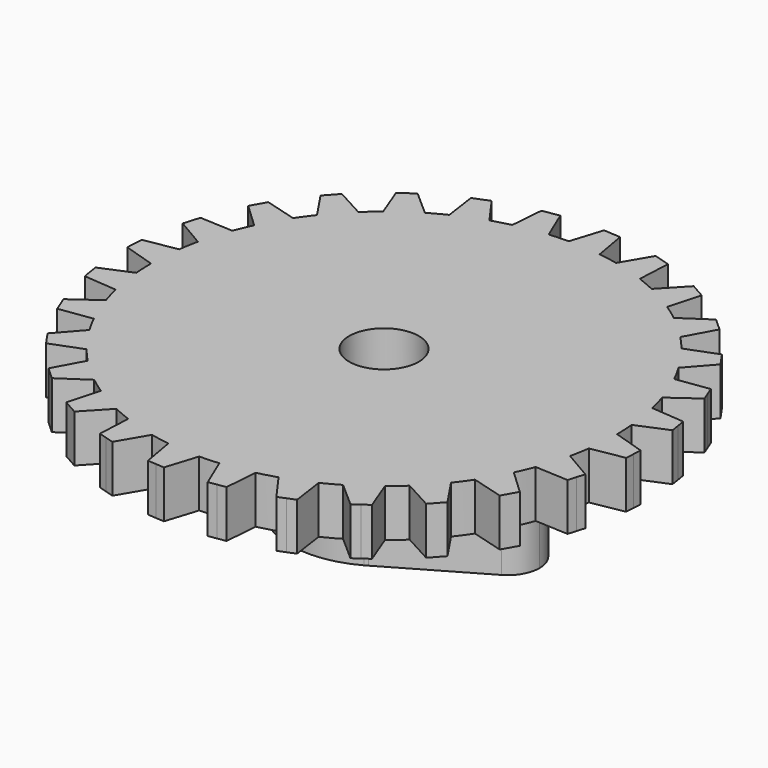
from build123d import *

# Parameters (mm, degrees)
F0_R     = 3.3
F1_DEPTH = 4.5
F2_DEPTH = 9
F4_COUNT = 28
F5_DEPTH = 9


# Not quite as in the source:
# - a feature names something its author has since deleted; it is built from what else it names


with BuildPart() as f1:
    # F0 (on Top) → F1 (new body)
    with BuildSketch(Plane.XY):
        with BuildLine():
            ThreePointArc((21.7954284513, -2.9932087503), (21.9487975289, -1.5000956754), (22, 0))
            ThreePointArc((22, 0), (21.9999455382, 0.0489521697), (21.9997821532, 0.097904097))
            ThreePointArc((21.9997821532, 0.097904097), (21.9765398394, 1.0157247108), (21.9150231618, 1.9317763373))
            ThreePointArc((21.9150231618, 1.9317763373), (21.7246308845, 3.4699298167), (21.426415972, 4.9908615085))
            ThreePointArc((21.426415972, 4.9908615085), (21.1995220913, 5.8804985418), (20.9357071018, 6.759894093))
            ThreePointArc((20.9357071018, 6.759894093), (20.4078170076, 8.2171165859), (19.778639825, 9.6335562839))
            ThreePointArc((19.778639825, 9.6335562839), (19.3594717841, 10.4503996211), (18.9065872678, 11.249042532))
            ThreePointArc((18.9065872678, 11.249042532), (18.0676699703, 12.5522628177), (17.1390800887, 13.793184321))
            ThreePointArc((17.1390800887, 13.793184321), (16.5486567235, 14.4962740264), (15.9294122011, 15.1741170065))
            ThreePointArc((15.9294122011, 15.1741170065), (14.8215345166, 16.2579861782), (13.6400953103, 17.2611645009))
            ThreePointArc((13.6400953103, 17.2611645009), (12.9080229136, 17.8152447208), (12.1534698913, 18.3382978927))
            ThreePointArc((12.1534698913, 18.3382978927), (10.832185433, 19.1484662243), (9.4571391969, 19.8635978164))
            ThreePointArc((9.4571391969, 19.8635978164), (8.6201269356, 20.2408846549), (7.7681018526, 20.5829199485))
            ThreePointArc((7.7681018526, 20.5829199485), (6.2996653405, 21.0787622169), (4.7999626346, 21.4699873942))
            ThreePointArc((4.7999626346, 21.4699873942), (3.8999817986, 21.6515621139), (2.9932087503, 21.7954284513))
            ThreePointArc((2.9932087503, 21.7954284513), (1.4512537227, 21.9520810547), (-0.097904097, 21.9997821532))
            ThreePointArc((-0.097904097, 21.9997821532), (-1.0157247108, 21.9765398394), (-1.9317763373, 21.9150231618))
            ThreePointArc((-1.9317763373, 21.9150231618), (-3.4699298167, 21.7246308845), (-4.9908615085, 21.426415972))
            ThreePointArc((-4.9908615085, 21.426415972), (-5.8804985418, 21.1995220913), (-6.759894093, 20.9357071018))
            ThreePointArc((-6.759894093, 20.9357071018), (-8.2171165859, 20.4078170076), (-9.6335562839, 19.778639825))
            ThreePointArc((-9.6335562839, 19.778639825), (-10.4503996211, 19.3594717841), (-11.249042532, 18.9065872678))
            ThreePointArc((-11.249042532, 18.9065872678), (-12.5522628177, 18.0676699703), (-13.793184321, 17.1390800887))
            ThreePointArc((-13.793184321, 17.1390800887), (-14.4962740264, 16.5486567235), (-15.1741170065, 15.9294122011))
            ThreePointArc((-15.1741170065, 15.9294122011), (-16.2579861782, 14.8215345166), (-17.2611645009, 13.6400953103))
            ThreePointArc((-17.2611645009, 13.6400953103), (-17.8152447208, 12.9080229136), (-18.3382978927, 12.1534698913))
            ThreePointArc((-18.3382978927, 12.1534698913), (-19.1484662243, 10.832185433), (-19.8635978164, 9.4571391969))
            ThreePointArc((-19.8635978164, 9.4571391969), (-20.2408846549, 8.6201269356), (-20.5829199485, 7.7681018526))
            ThreePointArc((-20.5829199485, 7.7681018526), (-21.0787622169, 6.2996653405), (-21.4699873942, 4.7999626346))
            ThreePointArc((-21.4699873942, 4.7999626346), (-21.6515621139, 3.8999817986), (-21.7954284513, 2.9932087503))
            ThreePointArc((-21.7954284513, 2.9932087503), (-21.9520810547, 1.4512537227), (-21.9997821532, -0.097904097))
            ThreePointArc((-21.9997821532, -0.097904097), (-21.9765398394, -1.0157247108), (-21.9150231618, -1.9317763373))
            ThreePointArc((-21.9150231618, -1.9317763373), (-21.7246308845, -3.4699298167), (-21.426415972, -4.9908615085))
            ThreePointArc((-21.426415972, -4.9908615085), (-21.1995220913, -5.8804985418), (-20.9357071018, -6.759894093))
            ThreePointArc((-20.9357071018, -6.759894093), (-20.4078170076, -8.2171165859), (-19.778639825, -9.6335562839))
            ThreePointArc((-19.778639825, -9.6335562839), (-19.3594717841, -10.4503996211), (-18.9065872678, -11.249042532))
            ThreePointArc((-18.9065872678, -11.249042532), (-18.0676699703, -12.5522628177), (-17.1390800887, -13.793184321))
            ThreePointArc((-17.1390800887, -13.793184321), (-16.5486567235, -14.4962740264), (-15.9294122011, -15.1741170065))
            ThreePointArc((-15.9294122011, -15.1741170065), (-14.8215345166, -16.2579861782), (-13.6400953103, -17.2611645009))
            ThreePointArc((-13.6400953103, -17.2611645009), (-12.9080229136, -17.8152447208), (-12.1534698913, -18.3382978927))
            ThreePointArc((-12.1534698913, -18.3382978927), (-10.832185433, -19.1484662243), (-9.4571391969, -19.8635978164))
            ThreePointArc((-9.4571391969, -19.8635978164), (-8.6201269356, -20.2408846549), (-7.7681018526, -20.5829199485))
            ThreePointArc((-7.7681018526, -20.5829199485), (-6.2996653405, -21.0787622169), (-4.7999626346, -21.4699873942))
            ThreePointArc((-4.7999626346, -21.4699873942), (-3.8999817986, -21.6515621139), (-2.9932087503, -21.7954284513))
            ThreePointArc((-2.9932087503, -21.7954284513), (-1.4512537227, -21.9520810547), (0.097904097, -21.9997821532))
            ThreePointArc((0.097904097, -21.9997821532), (1.0157247108, -21.9765398394), (1.9317763373, -21.9150231618))
            ThreePointArc((1.9317763373, -21.9150231618), (3.4699298167, -21.7246308845), (4.9908615085, -21.426415972))
            ThreePointArc((4.9908615085, -21.426415972), (5.8804985418, -21.1995220913), (6.759894093, -20.9357071018))
            ThreePointArc((6.759894093, -20.9357071018), (8.2171165859, -20.4078170076), (9.6335562839, -19.778639825))
            ThreePointArc((9.6335562839, -19.778639825), (10.4503996211, -19.3594717841), (11.249042532, -18.9065872678))
            ThreePointArc((11.249042532, -18.9065872678), (12.5522628177, -18.0676699703), (13.793184321, -17.1390800887))
            ThreePointArc((13.793184321, -17.1390800887), (14.4962740264, -16.5486567235), (15.1741170065, -15.9294122011))
            ThreePointArc((15.1741170065, -15.9294122011), (16.2579861782, -14.8215345166), (17.2611645009, -13.6400953103))
            ThreePointArc((17.2611645009, -13.6400953103), (17.8152447208, -12.9080229136), (18.3382978927, -12.1534698913))
            ThreePointArc((18.3382978927, -12.1534698913), (19.1484662243, -10.832185433), (19.8635978164, -9.4571391969))
            ThreePointArc((19.8635978164, -9.4571391969), (20.2408846549, -8.6201269356), (20.5829199485, -7.7681018526))
            ThreePointArc((20.5829199485, -7.7681018526), (21.0787622169, -6.2996653405), (21.4699873942, -4.7999626346))
            ThreePointArc((21.4699873942, -4.7999626346), (21.6515621139, -3.8999817986), (21.7954284513, -2.9932087503))
        make_face()
        with BuildLine():
            ThreePointArc((4.2957761194, -7.7649288031), (-8.8739963819, 0), (4.2957761194, 7.7649288031))
            ThreePointArc((4.2957761194, 7.7649288031), (4.4440805495, 7.6810129446), (4.5907463478, 7.5942649253))
            Line((4.5907463478, 7.5942649253), (13.2283979256, 2.5966923855))
            ThreePointArc((13.2283979256, 2.5966923855), (14.3247709146, 1.4988023682), (14.7260036181, 0))
            ThreePointArc((14.7260036181, 0), (14.3247709146, -1.4988023682), (13.2283979256, -2.5966923855))
            Line((13.2283979256, -2.5966923855), (4.5907463478, -7.5942649253))
            ThreePointArc((4.5907463478, -7.5942649253), (4.4440805495, -7.6810129446), (4.2957761194, -7.7649288031))
        make_face(mode=Mode.SUBTRACT)
        with BuildLine():
            Line((4.5907463478, 7.5942649253), (4.2957761194, 7.7649288031))
            ThreePointArc((4.2957761194, 7.7649288031), (-8.8739963819, 0), (4.2957761194, -7.7649288031))
            Line((4.2957761194, -7.7649288031), (4.5907463478, -7.5942649253))
            ThreePointArc((4.5907463478, -7.5942649253), (7.5224602815, -4.7074837333), (8.8370675717, -0.8087326625))
            ThreePointArc((8.8370675717, -0.8087326625), (8.7260036181, 0), (8.8370675717, 0.8087326625))
            ThreePointArc((8.8370675717, 0.8087326625), (7.5224602815, 4.7074837333), (4.5907463478, 7.5942649253))
        make_face()
        Circle(F0_R, mode=Mode.SUBTRACT)
        with BuildLine():
            Line((13.2283979256, 2.5966923855), (4.5907463478, 7.5942649253))
            ThreePointArc((4.5907463478, 7.5942649253), (7.5224602815, 4.7074837333), (8.8370675717, 0.8087326625))
            ThreePointArc((8.8370675717, 0.8087326625), (10.5947103355, 2.7785203812), (13.2283979256, 2.5966923855))
        make_face()
        with BuildLine():
            ThreePointArc((8.8370675717, -0.8087326625), (7.5224602815, -4.7074837333), (4.5907463478, -7.5942649253))
            Line((4.5907463478, -7.5942649253), (13.2283979256, -2.5966923855))
            ThreePointArc((13.2283979256, -2.5966923855), (10.5947103355, -2.7785203812), (8.8370675717, -0.8087326625))
        make_face()
        with BuildLine():
            ThreePointArc((-9.6335562839, 19.778639825), (-8.2171165859, 20.4078170076), (-6.759894093, 20.9357071018))
            Line((-6.759894093, 20.9357071018), (-8.5955300473, 23.4895053845))
            Line((-8.5955300473, 23.4895053845), (-9.3376324839, 23.190701145))
            Line((-9.3376324839, 23.190701145), (-10.0797349206, 22.8918969055))
            Line((-10.0797349206, 22.8918969055), (-9.6335562839, 19.778639825))
        make_face()
        with BuildLine():
            ThreePointArc((-17.2611645009, 13.6400953103), (-16.2579861782, 14.8215345166), (-15.1741170065, 15.9294122011))
            Line((-15.1741170065, 15.9294122011), (-17.936019402, 17.4338523572))
            Line((-17.936019402, 17.4338523572), (-18.4749842935, 16.8426528598))
            Line((-18.4749842935, 16.8426528598), (-19.013949185, 16.2514533624))
            Line((-19.013949185, 16.2514533624), (-17.2611645009, 13.6400953103))
        make_face()
        with BuildLine():
            ThreePointArc((17.1390800887, 13.793184321), (18.0676699703, 12.5522628177), (18.9065872678, 11.249042532))
            Line((18.9065872678, 11.249042532), (20.9878890687, 13.6069288394))
            Line((20.9878890687, 13.6069288394), (20.531443148, 14.2639350202))
            Line((20.531443148, 14.2639350202), (20.0749972274, 14.9209412009))
            Line((20.0749972274, 14.9209412009), (17.1390800887, 13.793184321))
        make_face()
        with BuildLine():
            ThreePointArc((-21.4699873942, 4.7999626346), (-21.0787622169, 6.2996653405), (-20.5829199485, 7.7681018526))
            Line((-20.5829199485, 7.7681018526), (-23.7240601432, 7.9252110584))
            Line((-23.7240601432, 7.9252110584), (-23.9531388829, 7.1587106142))
            Line((-23.9531388829, 7.1587106142), (-24.1822176225, 6.3922101699))
            Line((-24.1822176225, 6.3922101699), (-21.4699873942, 4.7999626346))
        make_face()
        with BuildLine():
            ThreePointArc((19.778639825, 9.6335562839), (20.4078170076, 8.2171165859), (20.9357071018, 6.759894093))
            Line((20.9357071018, 6.759894093), (23.4895053845, 8.5955300473))
            Line((23.4895053845, 8.5955300473), (23.190701145, 9.3376324839))
            Line((23.190701145, 9.3376324839), (22.8918969055, 10.0797349206))
            Line((22.8918969055, 10.0797349206), (19.778639825, 9.6335562839))
        make_face()
        with BuildLine():
            Line((-0.8508944647, -24.9983195157), (0.097904097, -21.9997821532))
            ThreePointArc((0.097904097, -21.9997821532), (-1.4512537227, -21.9520810547), (-2.9932087503, -21.7954284513))
            Line((-2.9932087503, -21.7954284513), (-2.4474094505, -24.8927737904))
            Line((-2.4474094505, -24.8927737904), (-1.6491519576, -24.9455466531))
            Line((-1.6491519576, -24.9455466531), (-0.8508944647, -24.9983195157))
        make_face()
        with BuildLine():
            ThreePointArc((21.426415972, 4.9908615085), (21.7246308845, 3.4699298167), (21.9150231618, 1.9317763373))
            Line((21.9150231618, 1.9317763373), (24.8132598166, 3.1531154868))
            Line((24.8132598166, 3.1531154868), (24.6870805506, 3.9431020644))
            Line((24.6870805506, 3.9431020644), (24.5609012845, 4.733088642))
            Line((24.5609012845, 4.733088642), (21.426415972, 4.9908615085))
        make_face()
        with BuildLine():
            Line((19.013949185, -16.2514533624), (17.2611645009, -13.6400953103))
            ThreePointArc((17.2611645009, -13.6400953103), (16.2579861782, -14.8215345166), (15.1741170065, -15.9294122011))
            Line((15.1741170065, -15.9294122011), (17.936019402, -17.4338523572))
            Line((17.936019402, -17.4338523572), (18.4749842935, -16.8426528598))
            Line((18.4749842935, -16.8426528598), (19.013949185, -16.2514533624))
        make_face()
        with BuildLine():
            Line((-20.0749972274, -14.9209412009), (-17.1390800887, -13.793184321))
            ThreePointArc((-17.1390800887, -13.793184321), (-18.0676699703, -12.5522628177), (-18.9065872678, -11.249042532))
            Line((-18.9065872678, -11.249042532), (-20.9878890687, -13.6069288394))
            Line((-20.9878890687, -13.6069288394), (-20.531443148, -14.2639350202))
            Line((-20.531443148, -14.2639350202), (-20.0749972274, -14.9209412009))
        make_face()
        with BuildLine():
            Line((-22.8918969055, -10.0797349206), (-19.778639825, -9.6335562839))
            ThreePointArc((-19.778639825, -9.6335562839), (-20.4078170076, -8.2171165859), (-20.9357071018, -6.759894093))
            Line((-20.9357071018, -6.759894093), (-23.4895053845, -8.5955300473))
            Line((-23.4895053845, -8.5955300473), (-23.190701145, -9.3376324839))
            Line((-23.190701145, -9.3376324839), (-22.8918969055, -10.0797349206))
        make_face()
        with BuildLine():
            Line((-24.5609012845, -4.733088642), (-21.426415972, -4.9908615085))
            ThreePointArc((-21.426415972, -4.9908615085), (-21.7246308845, -3.4699298167), (-21.9150231618, -1.9317763373))
            Line((-21.9150231618, -1.9317763373), (-24.8132598166, -3.1531154868))
            Line((-24.8132598166, -3.1531154868), (-24.6870805506, -3.9431020644))
            Line((-24.6870805506, -3.9431020644), (-24.5609012845, -4.733088642))
        make_face()
        with BuildLine():
            Line((-16.2514533624, -19.013949185), (-13.6400953103, -17.2611645009))
            ThreePointArc((-13.6400953103, -17.2611645009), (-14.8215345166, -16.2579861782), (-15.9294122011, -15.1741170065))
            Line((-15.9294122011, -15.1741170065), (-17.4338523572, -17.936019402))
            Line((-17.4338523572, -17.936019402), (-16.8426528598, -18.4749842935))
            Line((-16.8426528598, -18.4749842935), (-16.2514533624, -19.013949185))
        make_face()
        with BuildLine():
            ThreePointArc((-13.793184321, 17.1390800887), (-12.5522628177, 18.0676699703), (-11.249042532, 18.9065872678))
            Line((-11.249042532, 18.9065872678), (-13.6069288394, 20.9878890687))
            Line((-13.6069288394, 20.9878890687), (-14.2639350202, 20.531443148))
            Line((-14.2639350202, 20.531443148), (-14.9209412009, 20.0749972274))
            Line((-14.9209412009, 20.0749972274), (-13.793184321, 17.1390800887))
        make_face()
        with BuildLine():
            Line((-11.6129937657, -22.1535183616), (-9.4571391969, -19.8635978164))
            ThreePointArc((-9.4571391969, -19.8635978164), (-10.832185433, -19.1484662243), (-12.1534698913, -18.3382978927))
            Line((-12.1534698913, -18.3382978927), (-13.0056094911, -21.3657230574))
            Line((-13.0056094911, -21.3657230574), (-12.3093016284, -21.7596207095))
            Line((-12.3093016284, -21.7596207095), (-11.6129937657, -22.1535183616))
        make_face()
        with BuildLine():
            Line((14.9209412009, -20.0749972274), (13.793184321, -17.1390800887))
            ThreePointArc((13.793184321, -17.1390800887), (12.5522628177, -18.0676699703), (11.249042532, -18.9065872678))
            Line((11.249042532, -18.9065872678), (13.6069288394, -20.9878890687))
            Line((13.6069288394, -20.9878890687), (14.2639350202, -20.531443148))
            Line((14.2639350202, -20.531443148), (14.9209412009, -20.0749972274))
        make_face()
        with BuildLine():
            ThreePointArc((-21.9997821532, -0.097904097), (-21.9520810547, 1.4512537227), (-21.7954284513, 2.9932087503))
            Line((-21.7954284513, 2.9932087503), (-24.8927737904, 2.4474094505))
            Line((-24.8927737904, 2.4474094505), (-24.9455466531, 1.6491519576))
            Line((-24.9455466531, 1.6491519576), (-24.9983195157, 0.8508944647))
            Line((-24.9983195157, 0.8508944647), (-21.9997821532, -0.097904097))
        make_face()
        with BuildLine():
            ThreePointArc((13.6400953103, 17.2611645009), (14.8215345166, 16.2579861782), (15.9294122011, 15.1741170065))
            Line((15.9294122011, 15.1741170065), (17.4338523572, 17.936019402))
            Line((17.4338523572, 17.936019402), (16.8426528598, 18.4749842935))
            Line((16.8426528598, 18.4749842935), (16.2514533624, 19.013949185))
            Line((16.2514533624, 19.013949185), (13.6400953103, 17.2611645009))
        make_face()
        with BuildLine():
            Line((22.1535183616, -11.6129937657), (19.8635978164, -9.4571391969))
            ThreePointArc((19.8635978164, -9.4571391969), (19.1484662243, -10.832185433), (18.3382978927, -12.1534698913))
            Line((18.3382978927, -12.1534698913), (21.3657230574, -13.0056094911))
            Line((21.3657230574, -13.0056094911), (21.7596207095, -12.3093016284))
            Line((21.7596207095, -12.3093016284), (22.1535183616, -11.6129937657))
        make_face()
        with BuildLine():
            Line((4.733088642, -24.5609012845), (4.9908615085, -21.426415972))
            ThreePointArc((4.9908615085, -21.426415972), (3.4699298167, -21.7246308845), (1.9317763373, -21.9150231618))
            Line((1.9317763373, -21.9150231618), (3.1531154868, -24.8132598166))
            Line((3.1531154868, -24.8132598166), (3.9431020644, -24.6870805506))
            Line((3.9431020644, -24.6870805506), (4.733088642, -24.5609012845))
        make_face()
        with BuildLine():
            ThreePointArc((9.4571391969, 19.8635978164), (10.832185433, 19.1484662243), (12.1534698913, 18.3382978927))
            Line((12.1534698913, 18.3382978927), (13.0056094911, 21.3657230574))
            Line((13.0056094911, 21.3657230574), (12.3093016284, 21.7596207095))
            Line((12.3093016284, 21.7596207095), (11.6129937657, 22.1535183616))
            Line((11.6129937657, 22.1535183616), (9.4571391969, 19.8635978164))
        make_face()
        with BuildLine():
            ThreePointArc((4.7999626346, 21.4699873942), (6.2996653405, 21.0787622169), (7.7681018526, 20.5829199485))
            Line((7.7681018526, 20.5829199485), (7.9252110584, 23.7240601432))
            Line((7.9252110584, 23.7240601432), (7.1587106142, 23.9531388829))
            Line((7.1587106142, 23.9531388829), (6.3922101699, 24.1822176225))
            Line((6.3922101699, 24.1822176225), (4.7999626346, 21.4699873942))
        make_face()
        with BuildLine():
            ThreePointArc((-4.9908615085, 21.426415972), (-3.4699298167, 21.7246308845), (-1.9317763373, 21.9150231618))
            Line((-1.9317763373, 21.9150231618), (-3.1531154868, 24.8132598166))
            Line((-3.1531154868, 24.8132598166), (-3.9431020644, 24.6870805506))
            Line((-3.9431020644, 24.6870805506), (-4.733088642, 24.5609012845))
            Line((-4.733088642, 24.5609012845), (-4.9908615085, 21.426415972))
        make_face()
        with BuildLine():
            ThreePointArc((-19.8635978164, 9.4571391969), (-19.1484662243, 10.832185433), (-18.3382978927, 12.1534698913))
            Line((-18.3382978927, 12.1534698913), (-21.3657230574, 13.0056094911))
            Line((-21.3657230574, 13.0056094911), (-21.7596207095, 12.3093016284))
            Line((-21.7596207095, 12.3093016284), (-22.1535183616, 11.6129937657))
            Line((-22.1535183616, 11.6129937657), (-19.8635978164, 9.4571391969))
        make_face()
        with BuildLine():
            Line((10.0797349206, -22.8918969055), (9.6335562839, -19.778639825))
            ThreePointArc((9.6335562839, -19.778639825), (8.2171165859, -20.4078170076), (6.759894093, -20.9357071018))
            Line((6.759894093, -20.9357071018), (8.5955300473, -23.4895053845))
            Line((8.5955300473, -23.4895053845), (9.3376324839, -23.190701145))
            Line((9.3376324839, -23.190701145), (10.0797349206, -22.8918969055))
        make_face()
        with BuildLine():
            Line((-6.3922101699, -24.1822176225), (-4.7999626346, -21.4699873942))
            ThreePointArc((-4.7999626346, -21.4699873942), (-6.2996653405, -21.0787622169), (-7.7681018526, -20.5829199485))
            Line((-7.7681018526, -20.5829199485), (-7.9252110584, -23.7240601432))
            Line((-7.9252110584, -23.7240601432), (-7.1587106142, -23.9531388829))
            Line((-7.1587106142, -23.9531388829), (-6.3922101699, -24.1822176225))
        make_face()
        with BuildLine():
            ThreePointArc((-0.097904097, 21.9997821532), (1.4512537227, 21.9520810547), (2.9932087503, 21.7954284513))
            Line((2.9932087503, 21.7954284513), (2.4474094505, 24.8927737904))
            Line((2.4474094505, 24.8927737904), (1.6491519576, 24.9455466531))
            Line((1.6491519576, 24.9455466531), (0.8508944647, 24.9983195157))
            Line((0.8508944647, 24.9983195157), (-0.097904097, 21.9997821532))
        make_face()
        with BuildLine():
            ThreePointArc((21.9997821532, 0.097904097), (21.9999455382, 0.0489521697), (22, 0))
            ThreePointArc((22, 0), (21.9487975289, -1.5000956754), (21.7954284513, -2.9932087503))
            Line((21.7954284513, -2.9932087503), (24.8927737904, -2.4474094505))
            Line((24.8927737904, -2.4474094505), (24.9455466531, -1.6491519576))
            Line((24.9455466531, -1.6491519576), (24.9983195157, -0.8508944647))
            Line((24.9983195157, -0.8508944647), (21.9997821532, 0.097904097))
        make_face()
        with BuildLine():
            Line((24.1822176225, -6.3922101699), (21.4699873942, -4.7999626346))
            ThreePointArc((21.4699873942, -4.7999626346), (21.0787622169, -6.2996653405), (20.5829199485, -7.7681018526))
            Line((20.5829199485, -7.7681018526), (23.7240601432, -7.9252110584))
            Line((23.7240601432, -7.9252110584), (23.9531388829, -7.1587106142))
            Line((23.9531388829, -7.1587106142), (24.1822176225, -6.3922101699))
        make_face()
    extrude(amount=F1_DEPTH)


with BuildPart() as f2:
    # F0 (on Top) → F2 (new body)
    with BuildSketch(Plane.XY):
        with BuildLine():
            Line((13.2283979256, 2.5966923855), (4.5907463478, 7.5942649253))
            ThreePointArc((4.5907463478, 7.5942649253), (7.5224602815, 4.7074837333), (8.8370675717, 0.8087326625))
            ThreePointArc((8.8370675717, 0.8087326625), (10.5947103355, 2.7785203812), (13.2283979256, 2.5966923855))
        make_face()
        with BuildLine():
            ThreePointArc((8.8370675717, -0.8087326625), (7.5224602815, -4.7074837333), (4.5907463478, -7.5942649253))
            Line((4.5907463478, -7.5942649253), (13.2283979256, -2.5966923855))
            ThreePointArc((13.2283979256, -2.5966923855), (10.5947103355, -2.7785203812), (8.8370675717, -0.8087326625))
        make_face()
        with BuildLine():
            ThreePointArc((13.2283979256, 2.5966923855), (10.5947103355, 2.7785203812), (8.8370675717, 0.8087326625))
            ThreePointArc((8.8370675717, 0.8087326625), (8.8647593719, 0.4047876778), (8.8739963819, 0))
            ThreePointArc((8.8739963819, 0), (8.8647593719, -0.4047876778), (8.8370675717, -0.8087326625))
            ThreePointArc((8.8370675717, -0.8087326625), (10.5947103355, -2.7785203812), (13.2283979256, -2.5966923855))
            ThreePointArc((13.2283979256, -2.5966923855), (14.3247709146, -1.4988023682), (14.7260036181, 0))
            ThreePointArc((14.7260036181, 0), (14.3247709146, 1.4988023682), (13.2283979256, 2.5966923855))
        make_face()
        with BuildLine():
            ThreePointArc((8.8739963819, 0), (8.8647593719, 0.4047876778), (8.8370675717, 0.8087326625))
            ThreePointArc((8.8370675717, 0.8087326625), (8.7260036181, 0), (8.8370675717, -0.8087326625))
            ThreePointArc((8.8370675717, -0.8087326625), (8.8647593719, -0.4047876778), (8.8739963819, 0))
        make_face()
        with BuildLine():
            Line((4.5907463478, 7.5942649253), (4.2957761194, 7.7649288031))
            ThreePointArc((4.2957761194, 7.7649288031), (-8.8739963819, 0), (4.2957761194, -7.7649288031))
            Line((4.2957761194, -7.7649288031), (4.5907463478, -7.5942649253))
            ThreePointArc((4.5907463478, -7.5942649253), (7.5224602815, -4.7074837333), (8.8370675717, -0.8087326625))
            ThreePointArc((8.8370675717, -0.8087326625), (8.7260036181, 0), (8.8370675717, 0.8087326625))
            ThreePointArc((8.8370675717, 0.8087326625), (7.5224602815, 4.7074837333), (4.5907463478, 7.5942649253))
        make_face()
        Circle(F0_R, mode=Mode.SUBTRACT)
    extrude(amount=-F2_DEPTH)


with BuildPart() as f4_1:
    # F4: instance of F1
    add(f1.part.rotate(Axis((0, 0, 11.1139118671), (0, 0, 1)), 1 * 360 / F4_COUNT))


with BuildPart() as f4_2:
    # F4: instance of F1
    add(f1.part.rotate(Axis((0, 0, 11.1139118671), (0, 0, 1)), 2 * 360 / F4_COUNT))


with BuildPart() as f4_3:
    # F4: instance of F1
    add(f1.part.rotate(Axis((0, 0, 11.1139118671), (0, 0, 1)), 3 * 360 / F4_COUNT))


with BuildPart() as f4_4:
    # F4: instance of F1
    add(f1.part.rotate(Axis((0, 0, 11.1139118671), (0, 0, 1)), 4 * 360 / F4_COUNT))


with BuildPart() as f4_5:
    # F4: instance of F1
    add(f1.part.rotate(Axis((0, 0, 11.1139118671), (0, 0, 1)), 5 * 360 / F4_COUNT))


with BuildPart() as f4_6:
    # F4: instance of F1
    add(f1.part.rotate(Axis((0, 0, 11.1139118671), (0, 0, 1)), 6 * 360 / F4_COUNT))


with BuildPart() as f4_7:
    # F4: instance of F1
    add(f1.part.rotate(Axis((0, 0, 11.1139118671), (0, 0, 1)), 7 * 360 / F4_COUNT))


with BuildPart() as f4_8:
    # F4: instance of F1
    add(f1.part.rotate(Axis((0, 0, 11.1139118671), (0, 0, 1)), 8 * 360 / F4_COUNT))


with BuildPart() as f4_9:
    # F4: instance of F1
    add(f1.part.rotate(Axis((0, 0, 11.1139118671), (0, 0, 1)), 9 * 360 / F4_COUNT))


with BuildPart() as f4_10:
    # F4: instance of F1
    add(f1.part.rotate(Axis((0, 0, 11.1139118671), (0, 0, 1)), 10 * 360 / F4_COUNT))


with BuildPart() as f4_11:
    # F4: instance of F1
    add(f1.part.rotate(Axis((0, 0, 11.1139118671), (0, 0, 1)), 11 * 360 / F4_COUNT))


with BuildPart() as f4_12:
    # F4: instance of F1
    add(f1.part.rotate(Axis((0, 0, 11.1139118671), (0, 0, 1)), 12 * 360 / F4_COUNT))


with BuildPart() as f4_13:
    # F4: instance of F1
    add(f1.part.rotate(Axis((0, 0, 11.1139118671), (0, 0, 1)), 13 * 360 / F4_COUNT))


with BuildPart() as f4_14:
    # F4: instance of F1
    add(f1.part.rotate(Axis((0, 0, 11.1139118671), (0, 0, 1)), 14 * 360 / F4_COUNT))


with BuildPart() as f4_15:
    # F4: instance of F1
    add(f1.part.rotate(Axis((0, 0, 11.1139118671), (0, 0, 1)), 15 * 360 / F4_COUNT))


with BuildPart() as f4_16:
    # F4: instance of F1
    add(f1.part.rotate(Axis((0, 0, 11.1139118671), (0, 0, 1)), 16 * 360 / F4_COUNT))


with BuildPart() as f4_17:
    # F4: instance of F1
    add(f1.part.rotate(Axis((0, 0, 11.1139118671), (0, 0, 1)), 17 * 360 / F4_COUNT))


with BuildPart() as f4_18:
    # F4: instance of F1
    add(f1.part.rotate(Axis((0, 0, 11.1139118671), (0, 0, 1)), 18 * 360 / F4_COUNT))


with BuildPart() as f4_19:
    # F4: instance of F1
    add(f1.part.rotate(Axis((0, 0, 11.1139118671), (0, 0, 1)), 19 * 360 / F4_COUNT))


with BuildPart() as f4_20:
    # F4: instance of F1
    add(f1.part.rotate(Axis((0, 0, 11.1139118671), (0, 0, 1)), 20 * 360 / F4_COUNT))


with BuildPart() as f4_21:
    # F4: instance of F1
    add(f1.part.rotate(Axis((0, 0, 11.1139118671), (0, 0, 1)), 21 * 360 / F4_COUNT))


with BuildPart() as f4_22:
    # F4: instance of F1
    add(f1.part.rotate(Axis((0, 0, 11.1139118671), (0, 0, 1)), 22 * 360 / F4_COUNT))


with BuildPart() as f4_23:
    # F4: instance of F1
    add(f1.part.rotate(Axis((0, 0, 11.1139118671), (0, 0, 1)), 23 * 360 / F4_COUNT))


with BuildPart() as f4_24:
    # F4: instance of F1
    add(f1.part.rotate(Axis((0, 0, 11.1139118671), (0, 0, 1)), 24 * 360 / F4_COUNT))


with BuildPart() as f4_25:
    # F4: instance of F1
    add(f1.part.rotate(Axis((0, 0, 11.1139118671), (0, 0, 1)), 25 * 360 / F4_COUNT))


with BuildPart() as f4_26:
    # F4: instance of F1
    add(f1.part.rotate(Axis((0, 0, 11.1139118671), (0, 0, 1)), 26 * 360 / F4_COUNT))


with BuildPart() as f4_27:
    # F4: instance of F1
    add(f1.part.rotate(Axis((0, 0, 11.1139118671), (0, 0, 1)), 27 * 360 / F4_COUNT))


with BuildPart() as f1_1:
    add(f1.part)

    add(f2.part)  # F5 merges F2

    add(f4_1.part)  # F5 merges F4_1

    add(f4_2.part)  # F5 merges F4_2

    add(f4_3.part)  # F5 merges F4_3

    add(f4_4.part)  # F5 merges F4_4

    add(f4_5.part)  # F5 merges F4_5

    add(f4_6.part)  # F5 merges F4_6

    add(f4_7.part)  # F5 merges F4_7

    add(f4_8.part)  # F5 merges F4_8

    add(f4_9.part)  # F5 merges F4_9

    add(f4_10.part)  # F5 merges F4_10

    add(f4_11.part)  # F5 merges F4_11

    add(f4_12.part)  # F5 merges F4_12

    add(f4_13.part)  # F5 merges F4_13

    add(f4_14.part)  # F5 merges F4_14

    add(f4_15.part)  # F5 merges F4_15

    add(f4_16.part)  # F5 merges F4_16

    add(f4_17.part)  # F5 merges F4_17

    add(f4_18.part)  # F5 merges F4_18

    add(f4_19.part)  # F5 merges F4_19

    add(f4_20.part)  # F5 merges F4_20

    add(f4_21.part)  # F5 merges F4_21

    add(f4_22.part)  # F5 merges F4_22

    add(f4_23.part)  # F5 merges F4_23

    add(f4_24.part)  # F5 merges F4_24

    add(f4_25.part)  # F5 merges F4_25

    add(f4_26.part)  # F5 merges F4_26

    add(f4_27.part)  # F5 merges F4_27
    # F0 (on Top) → F5 (join)
    with BuildSketch(Plane.XY):
        with BuildLine():
            Line((4.5907463478, 7.5942649253), (4.2957761194, 7.7649288031))
            ThreePointArc((4.2957761194, 7.7649288031), (-8.8739963819, 0), (4.2957761194, -7.7649288031))
            Line((4.2957761194, -7.7649288031), (4.5907463478, -7.5942649253))
            ThreePointArc((4.5907463478, -7.5942649253), (7.5224602815, -4.7074837333), (8.8370675717, -0.8087326625))
            ThreePointArc((8.8370675717, -0.8087326625), (8.7260036181, 0), (8.8370675717, 0.8087326625))
            ThreePointArc((8.8370675717, 0.8087326625), (7.5224602815, 4.7074837333), (4.5907463478, 7.5942649253))
        make_face()
        Circle(F0_R, mode=Mode.SUBTRACT)
    extrude(amount=-F5_DEPTH)


solid = f1_1.part
